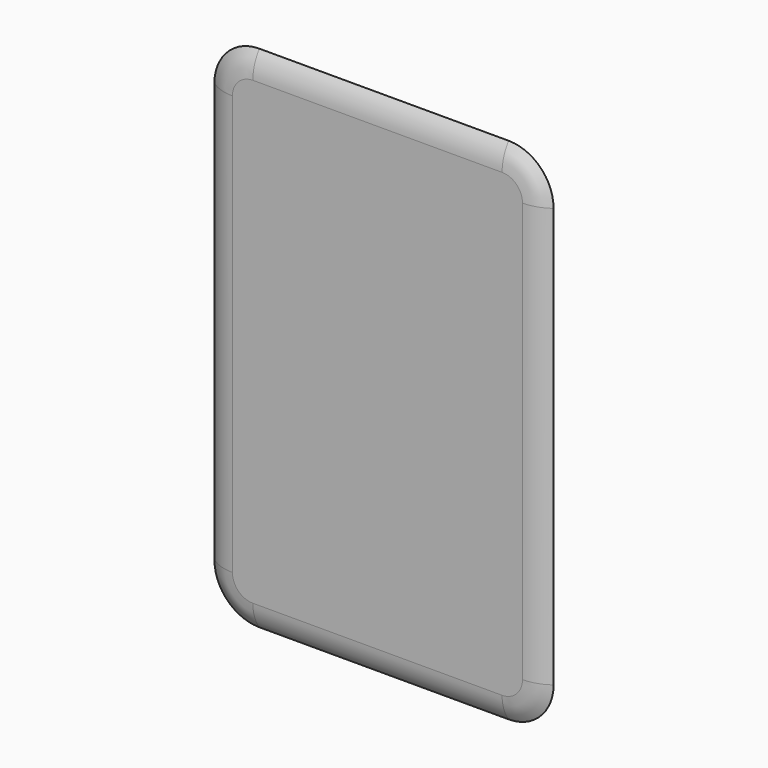
from build123d import *

# Parameters (mm, degrees)
F1_DEPTH     = 1.524
F2_T1_DEPTH  = 78.232
F2_T3_DEPTH  = 46.482
F2_T6_ANGLE  = 90
F2_T8_ANGLE  = 90
F2_T10_ANGLE = 90
F2_T12_ANGLE = 90


# Not quite as in the source:
# - a fillet or chamfer that OpenCascade refuses, or shapes differently, is made with other operations: its cross-section is extruded or revolved along the edge and cut away or added


with BuildPart() as f1:
    # F0 (on Front) → F1 (new body)
    with BuildSketch(Plane.XZ):
        with BuildLine():
            Line((-23.241, -47.498), (23.241, -47.498))
            ThreePointArc((23.241, -47.498), (29.1679690399, -45.0429690399), (31.623, -39.116))
            Line((31.623, -39.116), (31.623, 39.116))
            ThreePointArc((31.623, 39.116), (29.1679690399, 45.0429690399), (23.241, 47.498))
            Line((23.241, 47.498), (-23.241, 47.498))
            ThreePointArc((-23.241, 47.498), (-29.1679690399, 45.0429690399), (-31.623, 39.116))
            Line((-31.623, 39.116), (-31.623, -39.116))
            ThreePointArc((-31.623, -39.116), (-29.1679690399, -45.0429690399), (-23.241, -47.498))
        make_face()
    extrude(amount=F1_DEPTH)

    # F2: fillet of radius 7.62 on 1 edges, made by hand

    # F2_s2 → F2_t1 (cut)
    with BuildSketch(Plane.XY.offset(-39.116)):
        with BuildLine():
            ThreePointArc((-31.623, 0), (-29.460655577, -1.1329667311), (-27.051, -1.524))
            Line((-27.051, -1.524), (-31.623, -1.524))
            Line((-31.623, -1.524), (-31.623, 0))
        make_face()
        with BuildLine():
            ThreePointArc((31.623, 0), (29.460655577, -1.1329667311), (27.051, -1.524))
            Line((27.051, -1.524), (31.623, -1.524))
            Line((31.623, -1.524), (31.623, 0))
        make_face()
    extrude(amount=F2_T1_DEPTH, mode=Mode.SUBTRACT)

    # F2_s4 → F2_t3 (cut)
    with BuildSketch(Plane.YZ.offset(-23.241)):
        with BuildLine():
            ThreePointArc((0, -47.498), (-1.1329667311, -45.335655577), (-1.524, -42.926))
            Line((-1.524, -42.926), (-1.524, -47.498))
            Line((-1.524, -47.498), (0, -47.498))
        make_face()
        with BuildLine():
            ThreePointArc((0, 47.498), (-1.1329667311, 45.335655577), (-1.524, 42.926))
            Line((-1.524, 42.926), (-1.524, 47.498))
            Line((-1.524, 47.498), (0, 47.498))
        make_face()
    extrude(amount=F2_T3_DEPTH, mode=Mode.SUBTRACT)

    # F2_s5 → F2_t6 (revolve, cut)
    with BuildSketch(Plane.YZ.offset(-23.241)):
        with BuildLine():
            ThreePointArc((0, 47.498), (-1.1329667311, 45.335655577), (-1.524, 42.926))
            Line((-1.524, 42.926), (-1.524, 47.498))
            Line((-1.524, 47.498), (0, 47.498))
        make_face()
    revolve(axis=Axis((-23.241, -1.524, 39.116), (0, -1, 0)), revolution_arc=F2_T6_ANGLE, mode=Mode.SUBTRACT)

    # F2_s7 → F2_t8 (revolve, cut)
    with BuildSketch(Plane.XY.offset(-39.116)):
        with BuildLine():
            ThreePointArc((-31.623, 0), (-29.460655577, -1.1329667311), (-27.051, -1.524))
            Line((-27.051, -1.524), (-31.623, -1.524))
            Line((-31.623, -1.524), (-31.623, 0))
        make_face()
    revolve(axis=Axis((-23.241, -1.524, -39.116), (0, -1, 0)), revolution_arc=F2_T8_ANGLE, mode=Mode.SUBTRACT)

    # F2_s9 → F2_t10 (revolve, cut)
    with BuildSketch(Plane.YZ.offset(23.241)):
        with BuildLine():
            ThreePointArc((0, -47.498), (-1.1329667311, -45.335655577), (-1.524, -42.926))
            Line((-1.524, -42.926), (-1.524, -47.498))
            Line((-1.524, -47.498), (0, -47.498))
        make_face()
    revolve(axis=Axis((23.241, -1.524, -39.116), (0, -1, 0)), revolution_arc=F2_T10_ANGLE, mode=Mode.SUBTRACT)

    # F2_s11 → F2_t12 (revolve, cut)
    with BuildSketch(Plane.XY.offset(39.116)):
        with BuildLine():
            ThreePointArc((31.623, 0), (29.460655577, -1.1329667311), (27.051, -1.524))
            Line((27.051, -1.524), (31.623, -1.524))
            Line((31.623, -1.524), (31.623, 0))
        make_face()
    revolve(axis=Axis((23.241, -1.524, 39.116), (0, -1, 0)), revolution_arc=F2_T12_ANGLE, mode=Mode.SUBTRACT)


solid = f1.part
